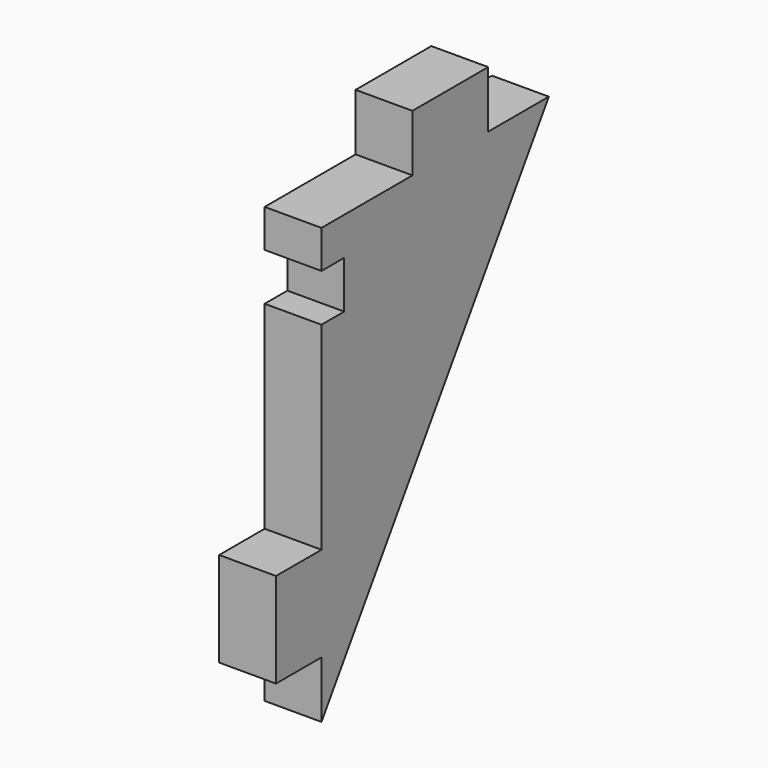
from build123d import *

# Parameters (mm, degrees)
F1_DEPTH = 3


# Not quite as in the source:
# - a feature names something its author has since deleted; it is built from what else it names


with BuildPart() as f1:
    # F0 (on Right) → F1 (new body)
    with BuildSketch(Plane.YZ):
        Polygon((-1.8767494946, 26.7287779992), (-7.8767494946, 26.7287779992), (-7.8767494946, 24.7287779992), (-6.3767494946, 24.7287779992), (-6.3767494946, 22.2287779992), (-7.8767494946, 22.2287779992), (-7.8767494946, 11.7737779992), (-10.8767494946, 11.7737779992), (-10.8767494946, 6.7737779992), (-7.8767494946, 6.7737779992), (-7.8767494946, 3.7737779992), (7.1232505054, 26.7287779992), (3.1232505054, 26.7287779992), (3.1232505054, 29.7287779992), (-1.8767494946, 29.7287779992), align=None)
    extrude(amount=F1_DEPTH)


solid = f1.part
